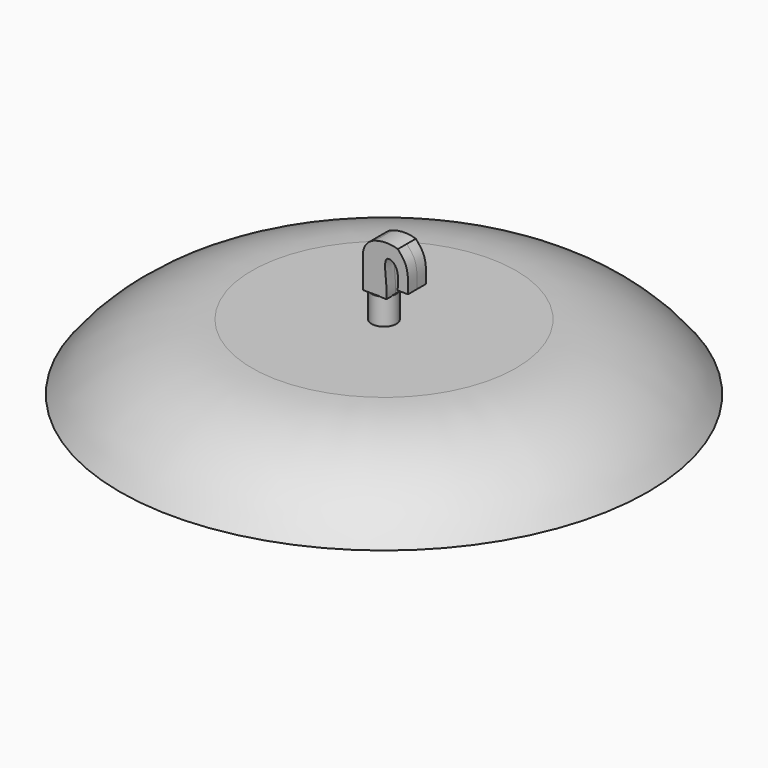
from build123d import *

# Parameters (mm, degrees)
F0_R     = 50.8
F1_DEPTH = 12.7
F4_R     = 2.3844019002
F5_DEPTH = 5.08
F7_DEPTH = 2.159
F8_R     = 46.183577677
F9_DEPTH = 4.318


# Not quite as in the source:
# - a fillet or chamfer that OpenCascade refuses, or shapes differently, is made with other operations: its cross-section is extruded or revolved along the edge and cut away or added


with BuildPart() as f1:
    # F0 (on Top) → F1 (new body)
    with BuildSketch(Plane.XY):
        Circle(F0_R)
    extrude(amount=F1_DEPTH)

    # F2: fillet of radius 31.75 on 1 edges, made by hand

    # F2_s1 → F2_t2 (revolve, cut)
    with BuildSketch(Plane.XZ):
        with BuildLine():
            ThreePointArc((50.8, 0), (39.5990316571, 9.3480633142), (25.4, 12.7))
            Line((25.4, 12.7), (50.8, 12.7))
            Line((50.8, 12.7), (50.8, 0))
        make_face()
    revolve(axis=Axis((0, 0, 12.7), (0, 0, 1)), mode=Mode.SUBTRACT)

    # F4 (on face) → F5 (join)
    with BuildSketch(Plane.XY.offset(12.7)):
        Circle(F4_R)
    extrude(amount=F5_DEPTH)

    # F6 (on Front) → F7 (join, symmetric)
    with BuildSketch(Plane.XZ):
        with BuildLine():
            Line((-2.3349747062, 23.7907841802), (-2.3349747062, 17.8023930639))
            Line((-2.3349747062, 17.8023930639), (2.1964372136, 17.6963582635))
            add(Edge.make_bspline(
                [(4.347205162, 19.8880601674), (4.4335474069, 20.8885193067), (4.5909606666, 22.7124852177), (3.6400970731, 24.6070794631), (1.4756871927, 24.9554852281), (2.3553322785, 19.8781417965), (2.2437732053, 18.3463361327), (2.1964372136, 17.6963582635)],
                knots=[0, 0, 0, 0, 0.2170343083, 0.395681564, 0.5347797532, 0.8025976366, 1, 1, 1, 1], degree=3))
            Line((4.347205162, 19.8880601674), (6.3592605293, 19.8880601674))
            add(Edge.make_bspline(
                [(4.3928744271, 26.9053261727), (5.0263463985, 26.1760936525), (6.4510931733, 24.5359710236), (6.3920513007, 21.5476896096), (6.3592605293, 19.8880601674)],
                knots=[0, 0, 0, 0, 0.4446207541, 1, 1, 1, 1], degree=3))
            ThreePointArc((4.3928744271, 26.9053261727), (2.1964372136, 27.2497590183), (0, 26.9053261727))
            ThreePointArc((0, 26.9053261727), (-1.6864120154, 25.7370934247), (-2.3349747062, 23.7907841802))
        make_face()
    extrude(amount=F7_DEPTH, both=True)

    # F8 (on face) → F9 (cut)
    with BuildSketch(Plane(origin=(0, 0, 0), x_dir=(1, 0, 0), z_dir=(0, 0, -1))):
        Circle(F8_R)
    extrude(amount=-F9_DEPTH, mode=Mode.SUBTRACT)


solid = f1.part
